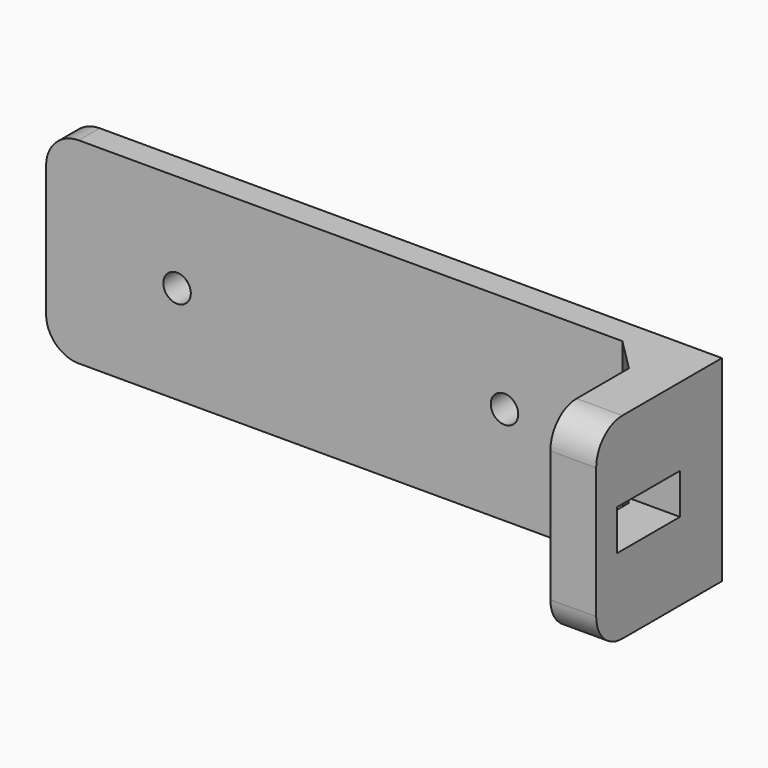
from build123d import *

# Parameters (mm, degrees)
F0_R     = 2.1
F1_DEPTH = 4
F2_W     = 7
F2_H     = 30
F3_DEPTH = 20
F5_W     = 5
F5_H     = 30
F6_DEPTH = 5
F7_SIZE  = 4.99999
F4_W     = 12
F4_H     = 6.2
F8_DEPTH = 10.8
F9_R     = 5


# Not quite as in the source:
# - a fillet or chamfer is up to 0.001 mm smaller than in the source, because OpenCascade refuses the exact size


with BuildPart() as f1:
    # F0 (on Front) → F1 (new body)
    with BuildSketch(Plane.XZ):
        with BuildLine():
            Line((55, 15), (-40, 15))
            ThreePointArc((-40, 15), (-43.5355339059, 13.5355339059), (-45, 10))
            Line((-45, 10), (-45, -10))
            ThreePointArc((-45, -10), (-43.5355339059, -13.5355339059), (-40, -15))
            Line((-40, -15), (55, -15))
            Line((55, -15), (55, 15))
        make_face()
        with Locations((-25, 0)):
            Circle(F0_R, mode=Mode.SUBTRACT)
        with Locations((25, 0)):
            Circle(F0_R, mode=Mode.SUBTRACT)
    extrude(amount=F1_DEPTH)

    # F2 (on face) → F3 (join)
    with BuildSketch(Plane.XZ.offset(4)):
        with Locations((51.5, 0)):
            Rectangle(F2_W, F2_H)
    extrude(amount=F3_DEPTH)

    # F5 (on face) → F6 (join)
    with BuildSketch(Plane.XZ.offset(4)):
        with Locations((45.5, 0)):
            Rectangle(F5_W, F5_H)
    extrude(amount=F6_DEPTH)

    # F7 (size 5 in the source; OpenCascade refuses exactly that, so slightly less here)
    f7_edges = [f1.edges().sort_by_distance(p)[0] for p in [
        (43, -9, 0),
    ]]
    chamfer(f7_edges, length=F7_SIZE)

    # F4 (on face) → F8 (cut, symmetric)
    with BuildSketch(Plane(origin=(48, 0, 0), x_dir=(0, -1, 0), z_dir=(-1, 0, 0))):
        with Locations((14, 0)):
            Rectangle(F4_W, F4_H)
    extrude(amount=F8_DEPTH, both=True, mode=Mode.SUBTRACT)

    # F9
    f9_edges = [f1.edges().sort_by_distance(p)[0] for p in [
        (51.5, -24, 15),
        (51.5, -24, -15),
    ]]
    fillet(f9_edges, radius=F9_R)


solid = f1.part
